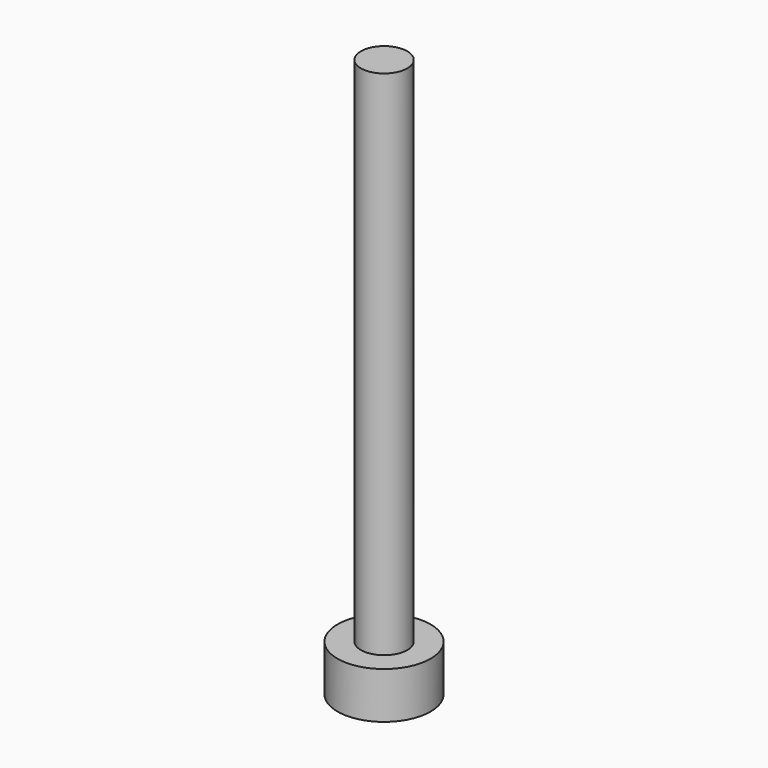
from build123d import *

# Parameters (mm, degrees)
F1_R     = 1.5812951981
F2_DEPTH = 34.925
F0_R     = 3.175
F3_DEPTH = 3.175
F5_DEPTH = 2.0052631579


# Not quite as in the source:
# - a length typed as a fraction of an inch, garbled in the dataset ("3 / 203.2 mm" for 3/8 in), is restored


with BuildPart() as f2:
    # F1 (on face) → F2 (new body)
    with BuildSketch(Plane.XY):
        with Locations((-0.0677817225, -10.2201197296)):
            Circle(F1_R)
    extrude(amount=F2_DEPTH)

    # F0 (on Top) → F3 (join)
    with BuildSketch(Plane.XY):
        with Locations((-0.0676529453, -10.2237053216)):
            Circle(F0_R)
    extrude(amount=-F3_DEPTH)

    # F4 (on face) → F5 (cut)
    with BuildSketch(Plane(origin=(0, 0, -3.175), x_dir=(1, 0, 0), z_dir=(0, 0, -1))):
        Polygon((-0.0660723406, 12.0567917448), (-1.6543620528, 11.141617377), (-1.6559426575, 9.3085309538), (-0.06923355, 8.3906188983), (1.5190561622, 9.3057932661), (1.5206367669, 11.1388796893), align=None)
    extrude(amount=-F5_DEPTH, mode=Mode.SUBTRACT)


solid = f2.part
